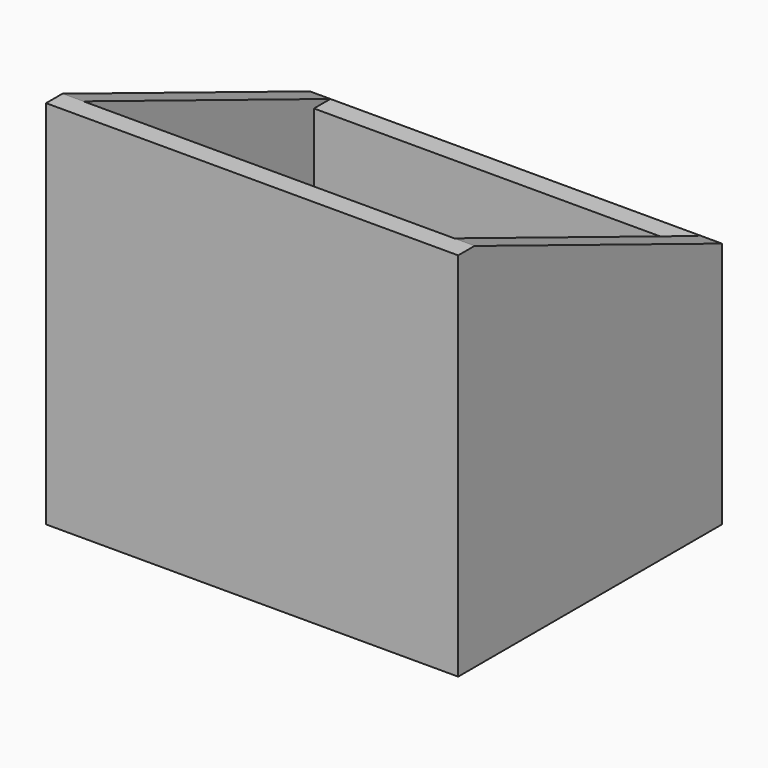
from build123d import *

# Parameters (mm, degrees)
F1_DEPTH = 60
F0_W     = 90
F0_H     = 70
F2_DEPTH = 10
F3_DEPTH = 90
F5_START = 45
F5_DEPTH = 5
F6_START = -45
F6_DEPTH = 5


with BuildPart() as f1:
    # F0 (on Top) → F1 (new body)
    with BuildSketch(Plane.XY):
        Polygon((45, -35), (50, -35), (50, 40), (-50, 40), (-50, -35), (-45, -35), (-45, 35), (45, 35), align=None)
    extrude(amount=F1_DEPTH)

    # F0 (on Top) → F2 (join)
    with BuildSketch(Plane.XY):
        Rectangle(F0_W, F0_H)
    extrude(amount=F2_DEPTH)

    # F0 (on Top) → F3 (join)
    with BuildSketch(Plane.XY):
        Polygon((-50, -40), (50, -40), (50, -35), (45, -35), (-45, -35), (-50, -35), align=None)
    extrude(amount=F3_DEPTH)

    # F4 (on Right) → F5 (join)
    with BuildSketch(Plane.YZ.offset(F5_START)):
        Polygon((-35.0263789296, 89.9869129062), (-35.307901961, 59.999383986), (39.9987436831, 59.999383986), align=None)
    extrude(amount=F5_DEPTH)

    # F4 (on Right) → F6 (join)
    with BuildSketch(Plane.YZ.offset(F6_START)):
        Polygon((-35.0263789296, 89.9869129062), (-35.307901961, 59.999383986), (39.9987436831, 59.999383986), align=None)
    extrude(amount=-F6_DEPTH)


solid = f1.part
